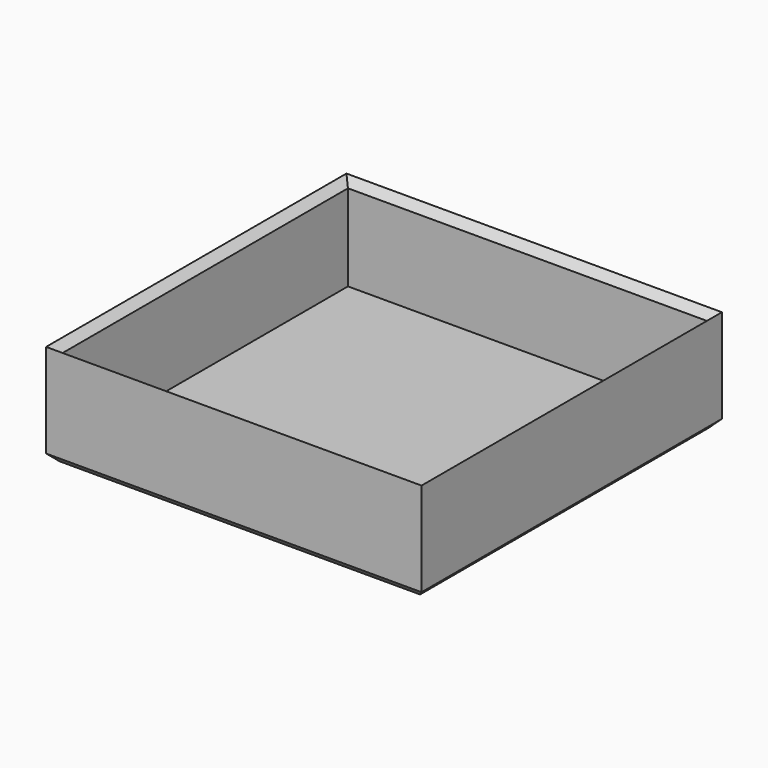
from build123d import *

# Parameters (mm, degrees)
F0_W     = 100
F0_H     = 100
F0_W_2   = 96
F0_H_2   = 96
F1_DEPTH = 25
F2_DEPTH = 2
F3_SIZE  = 1.99999


# Not quite as in the source:
# - a fillet or chamfer is up to 0.001 mm smaller than in the source, because OpenCascade refuses the exact size


with BuildPart() as f1:
    # F0 (on Top) → F1 (new body)
    with BuildSketch(Plane.XY):
        Rectangle(F0_W, F0_H)
        Rectangle(F0_W_2, F0_H_2, mode=Mode.SUBTRACT)
    extrude(amount=F1_DEPTH)

    # F0 (on Top) → F2 (join)
    with BuildSketch(Plane.XY):
        Rectangle(F0_W, F0_H)
        Rectangle(F0_W_2, F0_H_2, mode=Mode.SUBTRACT)
        Rectangle(F0_W_2, F0_H_2)
    extrude(amount=-F2_DEPTH)

    # F3 (size 2 in the source; OpenCascade refuses exactly that, so slightly less here)
    f3_edges = [f1.edges().sort_by_distance(p)[0] for p in [
        (0, -50, -2),
        (-50, 0, -2),
        (50, 0, -2),
        (0, 50, -2),
        (-48, 0, 25),
        (0, 48, 25),
        (48, 0, 25),
        (0, -48, 25),
    ]]
    chamfer(f3_edges, length=F3_SIZE)


solid = f1.part
